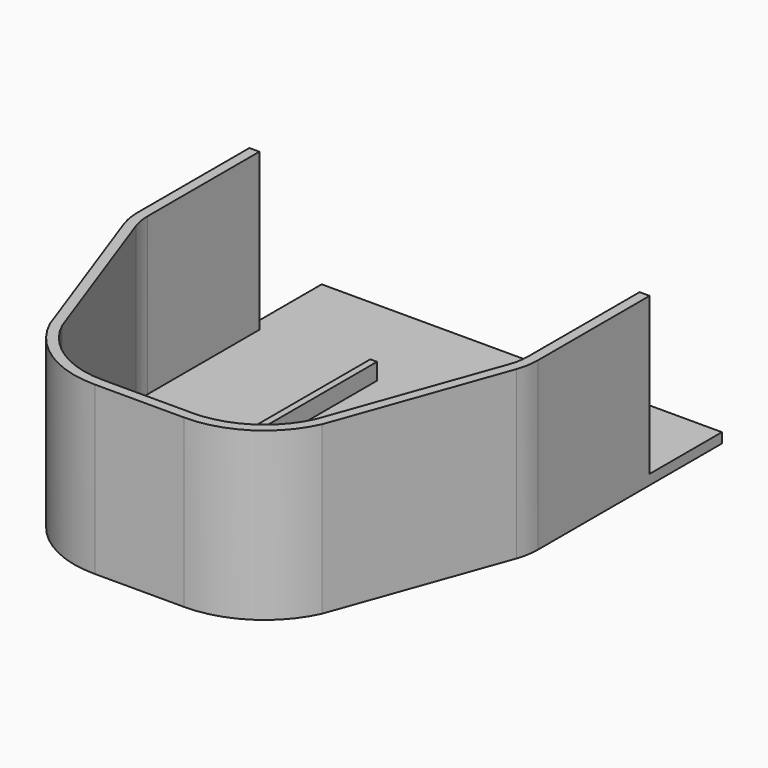
from build123d import *

# Parameters (mm, degrees)
F0_W     = 2
F0_H     = 85
F0_W_2   = 3.0000019335
F0_H_2   = 27.1
F1_DEPTH = 3
F2_DEPTH = 50
F3_DEPTH = 8


# Not quite as in the source:
# - ends of sketch curves that miss each other by under 0.0002 mm in the source are joined


with BuildPart() as f1:
    # F0 (on Top) → F1 (new body)
    with BuildSketch(Plane.XY):
        with BuildLine():
            Line((54.5097446937, 40.5472581927), (54.5097446937, 60.1075036168))
            Line((54.5097446937, 60.1075036168), (54.5097446937, 87.2075036168))
            Line((54.5097446937, 87.2075036168), (-59.4902514393, 87.2075036168))
            Line((-59.4902514393, 87.2075036168), (-59.4902514393, 60.1075036168))
            Line((-59.4902514393, 60.1075036168), (-59.4902514393, 40.5472581927))
            Line((-59.4902514393, 40.5472581927), (-59.4902514393, 18.2598339378))
            ThreePointArc((-59.4902514393, 18.2598339378), (-59.2538728212, 15.4347680531), (-58.5513104793, 12.6882651386))
            Line((-58.5513104793, 12.6882651386), (-40.5146915017, -37.5214353961))
            ThreePointArc((-40.5146915017, -37.5214353961), (-30.4754938788, -48.962906346), (-15.8429778585, -53.1560222908))
            Line((-15.8429778585, -53.1560222908), (10.8692885058, -53.1560668961))
            ThreePointArc((10.8692885058, -53.1560668961), (25.4978663276, -48.9610815315), (35.534184756, -37.5214353961))
            Line((35.534184756, -37.5214353961), (53.5708037336, 12.6882651386))
            ThreePointArc((53.5708037336, 12.6882651386), (54.2733660755, 15.4347680531), (54.5097446937, 18.2598339378))
            Line((54.5097446937, 18.2598339378), (54.5097446937, 40.5472581927))
        make_face()
        with Locations((-22.8452533728, 14.6164752861)):
            Rectangle(F0_W, F0_H, mode=Mode.SUBTRACT)
        with Locations((17.8647466272, 14.6164752861)):
            Rectangle(F0_W, F0_H, mode=Mode.SUBTRACT)
        with Locations((-60.9902524061, 73.6575036168)):
            Rectangle(F0_W_2, F0_H_2)
        with Locations((56.0097456604, 73.6575036168)):
            Rectangle(F0_W_2, F0_H_2)
    extrude(amount=F1_DEPTH)

    # F0 (on Top) → F2 (join)
    with BuildSketch(Plane.XY):
        with BuildLine():
            Line((-15.8404213062, -56.156068814), (10.8599145605, -56.1560242285))
            ThreePointArc((10.8599145605, -56.1560242285), (27.1664180437, -51.4552481906), (38.3132826454, -38.6588744882))
            Line((38.3132826454, -38.6588744882), (56.3994961696, 11.6888855872))
            ThreePointArc((56.3994961696, 11.6888855872), (57.2302307851, 14.9277918348), (57.5097466272, 18.2598339378))
            Line((57.5097466272, 18.2598339378), (57.5097466272, 40.2075055503))
            Line((57.5097466272, 40.2075055503), (57.5097466272, 60.1075036168))
            Line((57.5097466272, 60.1075036168), (54.5097446937, 60.1075036168))
            Line((54.5097446937, 60.1075036168), (54.5097446937, 40.5472581927))
            Line((54.5097446937, 40.5472581927), (54.5097446937, 18.2598339378))
            ThreePointArc((54.5097446937, 18.2598339378), (54.2733660755, 15.4347680531), (53.5708037336, 12.6882651386))
            Line((53.5708037336, 12.6882651386), (35.534184756, -37.5214353961))
            ThreePointArc((35.534184756, -37.5214353961), (25.4978663276, -48.9610815315), (10.8692885058, -53.1560668961))
            Line((10.8692885058, -53.1560668961), (-15.8429778585, -53.1560222908))
            ThreePointArc((-15.8429778585, -53.1560222908), (-30.4754938788, -48.962906346), (-40.5146915017, -37.5214353961))
            Line((-40.5146915017, -37.5214353961), (-58.5513104793, 12.6882651386))
            ThreePointArc((-58.5513104793, 12.6882651386), (-59.2538728212, 15.4347680531), (-59.4902514393, 18.2598339378))
            Line((-59.4902514393, 18.2598339378), (-59.4902514393, 40.5472581927))
            Line((-59.4902514393, 40.5472581927), (-59.4902514393, 60.1075036168))
            Line((-59.4902514393, 60.1075036168), (-62.4902533728, 60.1075036168))
            Line((-62.4902533728, 60.1075036168), (-62.4902533728, 40.2075055503))
            Line((-62.4902533728, 40.2075055503), (-62.4902533728, 18.2598339378))
            ThreePointArc((-62.4902533728, 18.2598339378), (-62.2107375308, 14.9277918348), (-61.3800029152, 11.6888855872))
            Line((-61.3800029152, 11.6888855872), (-43.293789391, -38.6588744882))
            ThreePointArc((-43.293789391, -38.6588744882), (-32.1469247894, -51.4552481906), (-15.8404213062, -56.156068814))
        make_face()
    extrude(amount=F2_DEPTH)

    # F0 (on Top) → F3 (join)
    with BuildSketch(Plane.XY):
        with Locations((17.8647466272, 14.6164752861)):
            Rectangle(F0_W, F0_H)
        with Locations((-22.8452533728, 14.6164752861)):
            Rectangle(F0_W, F0_H)
    extrude(amount=F3_DEPTH)


solid = f1.part
